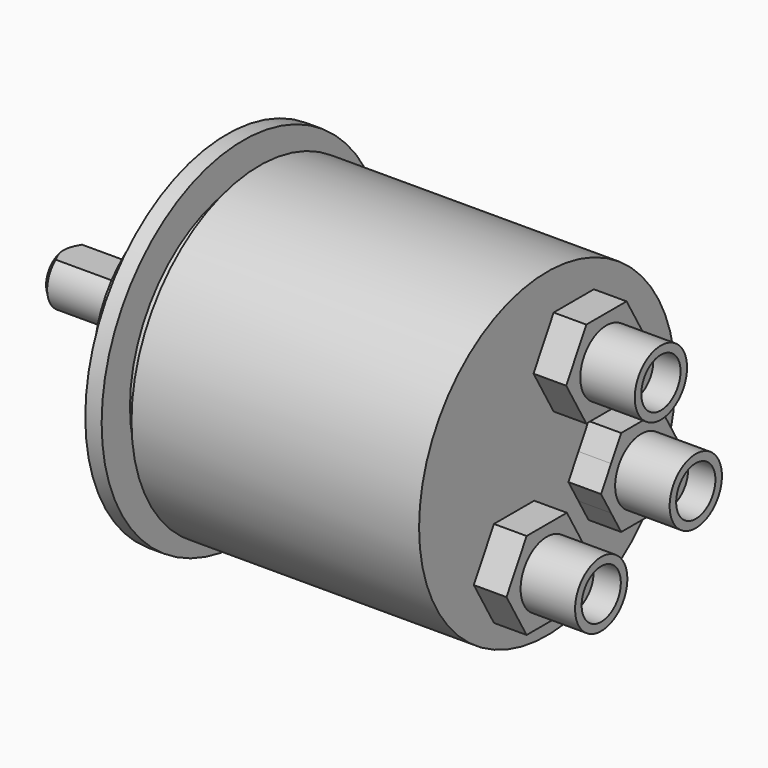
from build123d import *

# Parameters (mm, degrees)
F0_R        = 5
F1_DEPTH    = 18.9
F2_W        = 21.1690347642
F2_H        = 4.931249544
F3_DEPTH    = 18.901
F4_T2_ANGLE = 359.64
F5_R        = 7
F6_DEPTH    = 1.1
F7_R        = 18
F8_DEPTH    = 10
F9_R        = 32.5
F10_DEPTH   = 3
F11_R       = 26
F12_DEPTH   = 3
F14_R       = 29.4
F15_DEPTH   = 52.8
F16_R       = 1.75
F17_DEPTH   = 3
F19_DEPTH   = 6
F20_R       = 6
F21_DEPTH   = 10
F22_R       = 4.5
F23_DEPTH   = 5


# Not quite as in the source:
# - a fillet or chamfer that OpenCascade refuses, or shapes differently, is made with other operations: its cross-section is extruded or revolved along the edge and cut away or added


with BuildPart() as f1:
    # F0 (on Right) → F1 (new body)
    with BuildSketch(Plane.YZ):
        Circle(F0_R)
    extrude(amount=-F1_DEPTH)

    # F2 (on Right) → F3 (cut, through all)
    with BuildSketch(Plane.YZ):
        with Locations((0.0764410943, 6.465624772)):
            Rectangle(F2_W, F2_H)
    extrude(amount=-F3_DEPTH, mode=Mode.SUBTRACT)

    # F4: chamfer of 1 on 1 edges, made by hand

    # F4_s1 → F4_t2 (revolve, cut)
    with BuildSketch(Plane(origin=(0, 0, 0), x_dir=(1, 0, 0), z_dir=(0, 0.9999950652, 0.0031415875))):
        with BuildLine():
            Line((-17.8717157288, -5.0282842712), (-18.9282842712, -3.9717157288))
            Line((-18.9282842712, -3.9717157288), (-18.9482842712, -3.9717157288))
            ThreePointArc((-18.9482842712, -3.9717157288), (-18.92, -4.4858578644), (-18.92, -5))
            Line((-18.92, -5), (-18.9, -5.02))
            ThreePointArc((-18.9, -5.02), (-18.3858578644, -5.02), (-17.8717157288, -5.0482842712))
            Line((-17.8717157288, -5.0482842712), (-17.8717157288, -5.0282842712))
        make_face()
    revolve(axis=Axis((-18.9, 0, 0), (1, 0, 0)), revolution_arc=F4_T2_ANGLE, mode=Mode.SUBTRACT)

    # F5 (on face) → F6 (join)
    with BuildSketch(Plane.YZ):
        Circle(F5_R)
    extrude(amount=F6_DEPTH)

    # F7 (on face) → F8 (join)
    with BuildSketch(Plane.YZ.offset(1.1)):
        Circle(F7_R)
    extrude(amount=F8_DEPTH)

    # F9 (on face) → F10 (join)
    with BuildSketch(Plane.YZ.offset(11.1)):
        Circle(F9_R)
    extrude(amount=F10_DEPTH)

    # F11 (on face) → F12 (join)
    with BuildSketch(Plane.YZ.offset(14.1)):
        Circle(F11_R)
    extrude(amount=F12_DEPTH)

    # F14 (on offset) → F15 (join, through all)
    with BuildSketch(Plane(origin=(69.9, 0, 0), x_dir=(0, -1, 0), z_dir=(-1, 0, 0))):
        Circle(F14_R)
    extrude(amount=F15_DEPTH)

    # F16 (on face) → F17 (cut)
    with BuildSketch(Plane(origin=(11.1, 0, 0), x_dir=(0, -1, 0), z_dir=(-1, 0, 0))):
        with Locations((-24, 0)):
            Circle(F16_R)
        with Locations((12, -20.7846096908)):
            Circle(F16_R)
        with Locations((12, 20.7846096908)):
            Circle(F16_R)
    extrude(amount=-F17_DEPTH, mode=Mode.SUBTRACT)

    # F18 (on face) → F19 (join)
    with BuildSketch(Plane.YZ.offset(69.9)):
        with BuildLine():
            ThreePointArc((21.0282031968, -10.574938038), (21.8274066017, -8.6454903731), (22.1, -6.57493798))
            ThreePointArc((22.1, -6.57493798), (21.8274066078, -4.5043856099), (21.0282032207, -2.5749379634))
            ThreePointArc((21.0282032207, -2.5749379634), (18.0999999917, 0.3532652551), (14.1, 1.42506202))
            ThreePointArc((14.1, 1.42506202), (10.1000001451, 0.3532653341), (7.1717969373, -2.5749376897))
            ThreePointArc((7.1717969373, -2.5749376897), (6.1, -6.5749379695), (7.1717969269, -10.5749382522))
            ThreePointArc((7.1717969269, -10.5749382522), (10.1000001361, -13.5031412888), (14.1, -14.57493798))
            ThreePointArc((14.1, -14.57493798), (18.099999971, -13.503141227), (21.0282031968, -10.574938038))
        make_face()
        with BuildLine():
            ThreePointArc((21.0282032207, -2.5749379634), (21.8274066078, -4.5043856099), (22.1, -6.57493798))
            ThreePointArc((22.1, -6.57493798), (21.8274066017, -8.6454903731), (21.0282031968, -10.574938038))
            Line((21.0282031968, -10.574938038), (23.337604307, -6.57493798))
            Line((23.337604307, -6.57493798), (21.0282032207, -2.5749379634))
        make_face()
        with BuildLine():
            ThreePointArc((14.1, 1.42506202), (18.0999999917, 0.3532652551), (21.0282032207, -2.5749379634))
            Line((21.0282032207, -2.5749379634), (18.7188021535, 1.42506202))
            Line((18.7188021535, 1.42506202), (14.1, 1.42506202))
        make_face()
        with BuildLine():
            Line((18.7188021535, -14.57493798), (21.0282031968, -10.574938038))
            ThreePointArc((21.0282031968, -10.574938038), (18.099999971, -13.503141227), (14.1, -14.57493798))
            Line((14.1, -14.57493798), (18.7188021535, -14.57493798))
        make_face()
        with BuildLine():
            ThreePointArc((7.1717969373, -2.5749376897), (10.1000001451, 0.3532653341), (14.1, 1.42506202))
            Line((14.1, 1.42506202), (9.4811978465, 1.42506202))
            Line((9.4811978465, 1.42506202), (7.1717969373, -2.5749376897))
        make_face()
        with BuildLine():
            Line((9.4811978465, -14.57493798), (14.1, -14.57493798))
            ThreePointArc((14.1, -14.57493798), (10.1000001361, -13.5031412888), (7.1717969269, -10.5749382522))
            Line((7.1717969269, -10.5749382522), (9.4811978465, -14.57493798))
        make_face()
        with BuildLine():
            ThreePointArc((7.1717969269, -10.5749382522), (6.1, -6.5749379695), (7.1717969373, -2.5749376897))
            Line((7.1717969373, -2.5749376897), (4.862395693, -6.57493798))
            Line((4.862395693, -6.57493798), (7.1717969269, -10.5749382522))
        make_face()
        Polygon((10.7188021535, 22.2), (1.4811978465, 22.2), (-3.137604307, 14.2), (1.4811978465, 6.2), (10.7188021535, 6.2), (15.337604307, 14.2), align=None)
        Polygon((-2.9811978465, -6.4), (-12.2188021535, -6.4), (-16.837604307, -14.4), (-12.2188021535, -22.4), (-2.9811978465, -22.4), (1.637604307, -14.4), align=None)
    extrude(amount=F19_DEPTH)

    # F20 (on face) → F21 (join)
    with BuildSketch(Plane.YZ.offset(75.9)):
        with Locations((6.1, 14.2)):
            Circle(F20_R)
        with Locations((14.1, -6.57493798)):
            Circle(F20_R)
        with Locations((-7.6, -14.4)):
            Circle(F20_R)
    extrude(amount=F21_DEPTH)

    # F22 (on face) → F23 (cut)
    with BuildSketch(Plane.YZ.offset(85.9)):
        with Locations((6.1, 14.2)):
            Circle(F22_R)
        with Locations((-7.6, -14.4)):
            Circle(F22_R)
        with Locations((14.1, -6.57493798)):
            Circle(F22_R)
    extrude(amount=-F23_DEPTH, mode=Mode.SUBTRACT)


solid = f1.part
